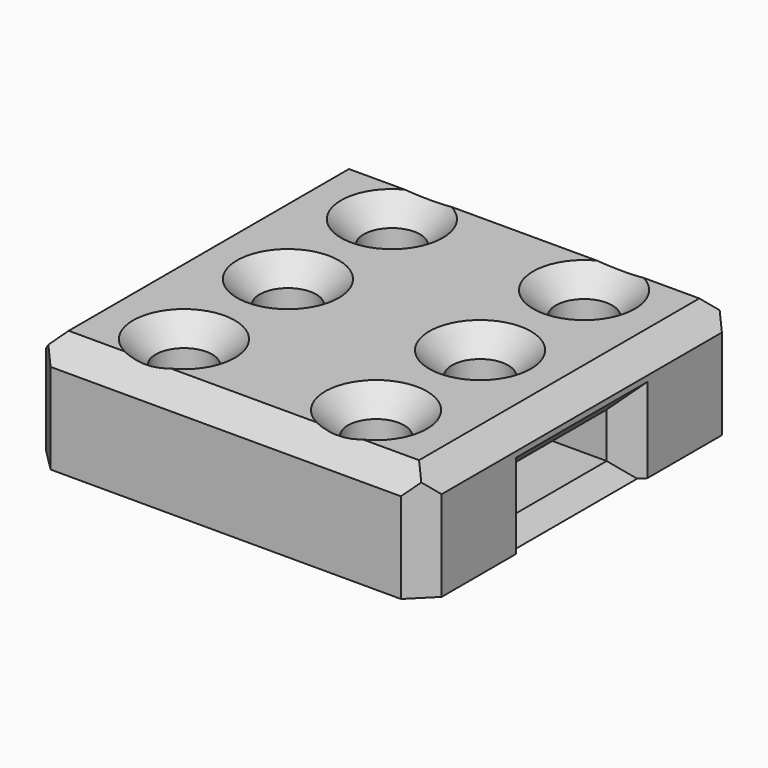
from build123d import *

# Parameters (mm, degrees)
F0_W          = 44.45
F0_H          = 44.45
F1_DEPTH      = 12.7
F2_W          = 13.335
F2_H          = 5.08
F3_DEPTH      = 76.2
F4_R          = 3.175
F5_DEPTH      = 25.4
F6_T1_DEPTH   = 57.5141495789
F6_T3_DEPTH   = 57.5141495789
F7_T1_DEPTH   = 5.08
F7_T3_DEPTH   = 13.335
F7_T5_DEPTH   = 23.2241495789
F7_T11_DEPTH  = 19.8670747894
F7_T16_DEPTH  = 11.6120747894
F7_T24_DEPTH  = 19.8670747894
F7_T28_DEPTH  = 11.6120747894
F7_T36_DEPTH  = 11.6120747894
F7_T41_DEPTH  = 19.8670747894
F7_T49_DEPTH  = 11.6120747894
F7_T54_DEPTH  = 19.8670747894
F7_T61_DEPTH  = 19.8670747894
F7_T65_DEPTH  = 11.6120747894
F7_T73_DEPTH  = 11.6120747894
F7_T78_DEPTH  = 19.8670747894
F7_T85_DEPTH  = 19.8670747894
F7_T90_DEPTH  = 11.6120747894
F7_T98_DEPTH  = 11.6120747894
F7_T103_DEPTH = 19.8670747894
F8_R          = 3.175
F9_DEPTH      = 1.905


# Not quite as in the source:
# - a fillet or chamfer that OpenCascade refuses, or shapes differently, is made with other operations: its cross-section is extruded or revolved along the edge and cut away or added


with BuildPart() as f1:
    # F0 (on Top) → F1 (new body)
    with BuildSketch(Plane.XY):
        Rectangle(F0_W, F0_H)
    extrude(amount=F1_DEPTH)

    # F2 (on face) → F3 (cut)
    with BuildSketch(Plane.YZ.offset(22.225)):
        with Locations((0, 4.445)):
            Rectangle(F2_W, F2_H)
    extrude(amount=-F3_DEPTH, mode=Mode.SUBTRACT)

    # F4 (on face) → F5 (cut)
    with BuildSketch(Plane.XY.offset(12.7)):
        with Locations((10.795, 14.605)):
            Circle(F4_R)
        with Locations((-10.795, 14.605)):
            Circle(F4_R)
        with Locations((-10.795, -14.605)):
            Circle(F4_R)
        with Locations((10.795, -14.605)):
            Circle(F4_R)
        with Locations((-10.795, 0)):
            Circle(F4_R)
        with Locations((10.795, 0)):
            Circle(F4_R)
    extrude(amount=-F5_DEPTH, mode=Mode.SUBTRACT)

    # F6: chamfer of 2.54 on 10 edges, made by hand

    # F6_s2 → F6_t1 (cut)
    with BuildSketch(Plane.XZ.offset(-28.7570747894)):
        Polygon((22.225, 10.16), (19.685, 12.7), (22.225, 12.7), align=None)
        Polygon((-19.685, 12.7), (-22.225, 10.16), (-22.225, 12.7), align=None)
    extrude(amount=F6_T1_DEPTH, mode=Mode.SUBTRACT)

    # F6_s4 → F6_t3 (cut)
    with BuildSketch(Plane.YZ.offset(-28.7570747894)):
        Polygon((-22.225, 10.16), (-19.685, 12.7), (-22.225, 12.7), align=None)
        Polygon((19.685, 12.7), (22.225, 10.16), (22.225, 12.7), align=None)
    extrude(amount=F6_T3_DEPTH, mode=Mode.SUBTRACT)

    # F6_s5 → F6_t6 (revolve, cut)
    with BuildSketch(Plane.XZ.offset(14.605)):
        Polygon((-5.08, 12.7), (-7.62, 10.16), (-7.62, 12.7), align=None)
    revolve(axis=Axis((-10.795, -14.605, 12.7), (0, 0, 1)), mode=Mode.SUBTRACT)

    # F6_s7 → F6_t8 (revolve, cut)
    with BuildSketch(Plane.XZ):
        Polygon((-5.08, 12.7), (-7.62, 10.16), (-7.62, 12.7), align=None)
    revolve(axis=Axis((-10.795, 0, 12.7), (0, 0, 1)), mode=Mode.SUBTRACT)

    # F6_s9 → F6_t10 (revolve, cut)
    with BuildSketch(Plane.XZ.offset(14.605)):
        Polygon((16.51, 12.7), (13.97, 10.16), (13.97, 12.7), align=None)
    revolve(axis=Axis((10.795, -14.605, 12.7), (0, 0, 1)), mode=Mode.SUBTRACT)

    # F6_s11 → F6_t12 (revolve, cut)
    with BuildSketch(Plane.XZ):
        Polygon((16.51, 12.7), (13.97, 10.16), (13.97, 12.7), align=None)
    revolve(axis=Axis((10.795, 0, 12.7), (0, 0, 1)), mode=Mode.SUBTRACT)

    # F6_s13 → F6_t14 (revolve, cut)
    with BuildSketch(Plane.XZ.offset(-14.605)):
        Polygon((-5.08, 12.7), (-7.62, 10.16), (-7.62, 12.7), align=None)
    revolve(axis=Axis((-10.795, 14.605, 12.7), (0, 0, 1)), mode=Mode.SUBTRACT)

    # F6_s15 → F6_t16 (revolve, cut)
    with BuildSketch(Plane.XZ.offset(-14.605)):
        Polygon((16.51, 12.7), (13.97, 10.16), (13.97, 12.7), align=None)
    revolve(axis=Axis((10.795, 14.605, 12.7), (0, 0, 1)), mode=Mode.SUBTRACT)

    # F7: chamfer of 2.54 on 12 edges, made by hand

    # F7_s2 → F7_t1 (cut)
    with BuildSketch(Plane.XY.offset(1.905)):
        Polygon((22.225, 9.2075), (19.685, 6.6675), (22.225, 6.6675), align=None)
        Polygon((22.225, -9.2075), (19.685, -6.6675), (22.225, -6.6675), align=None)
        Polygon((-19.685, 6.6675), (-22.225, 9.2075), (-22.225, 6.6675), align=None)
        Polygon((-19.685, -6.6675), (-22.225, -9.2075), (-22.225, -6.6675), align=None)
    extrude(amount=F7_T1_DEPTH, mode=Mode.SUBTRACT)

    # F7_s4 → F7_t3 (cut)
    with BuildSketch(Plane.XZ.offset(-6.6675)):
        Polygon((22.225, -0.635), (19.685, 1.905), (22.225, 1.905), align=None)
        Polygon((22.225, 9.525), (19.685, 6.985), (22.225, 6.985), align=None)
        Polygon((-19.685, 6.985), (-22.225, 9.525), (-22.225, 6.985), align=None)
        Polygon((-19.685, 1.905), (-22.225, -0.635), (-22.225, 1.905), align=None)
    extrude(amount=F7_T3_DEPTH, mode=Mode.SUBTRACT)

    # F7_s6 → F7_t5 (cut)
    with BuildSketch(Plane.XY.offset(-6.5320747894)):
        Polygon((-19.685, -22.225), (-22.225, -19.685), (-22.225, -22.225), align=None)
        Polygon((22.225, -19.685), (19.685, -22.225), (22.225, -22.225), align=None)
        Polygon((22.225, 19.685), (19.685, 22.225), (22.225, 22.225), align=None)
        Polygon((-19.685, 22.225), (-22.225, 19.685), (-22.225, 22.225), align=None)
    extrude(amount=F7_T5_DEPTH, mode=Mode.SUBTRACT)


with BuildPart() as f7_tool9:
    # F7_s10 → F7_t11 (new body)
    with BuildSketch(Plane.XZ.offset(6.6675)):
        Polygon((22.225, -0.635), (19.685, 1.905), (22.225, 1.905), align=None)
    extrude(amount=-F7_T11_DEPTH)

    split(bisect_by=Plane.XY, keep=Keep.TOP)

    split(bisect_by=Plane.XZ.offset(-6.6675), keep=Keep.BOTTOM)


with BuildPart() as f7_tool14:
    # F7_s15 → F7_t16 (new body)
    with BuildSketch(Plane.XY.offset(-4.6270747894)):
        Polygon((22.225, 9.2075), (19.685, 6.6675), (22.225, 6.6675), align=None)
    extrude(amount=F7_T16_DEPTH)

    split(bisect_by=Plane.XY, keep=Keep.TOP)

    split(bisect_by=Plane.XY.offset(1.905), keep=Keep.BOTTOM)


with BuildPart() as f7_tool9_1:
    add(f7_tool9.part)

    # F7_t19: intersect F7_tool14
    add(f7_tool14.part, mode=Mode.INTERSECT)


with BuildPart() as f1_1:
    add(f1.part)

    # F7_t7: cut F7_tool9
    add(f7_tool9_1.part, mode=Mode.SUBTRACT)


with BuildPart() as f7_tool22:
    # F7_s23 → F7_t24 (new body)
    with BuildSketch(Plane.XZ.offset(-13.1995747894)):
        Polygon((22.225, 9.525), (19.685, 6.985), (22.225, 6.985), align=None)
    extrude(amount=F7_T24_DEPTH)

    split(bisect_by=Plane.XZ.offset(-6.6675), keep=Keep.BOTTOM)


with BuildPart() as f7_tool26:
    # F7_s27 → F7_t28 (new body)
    with BuildSketch(Plane.XY.offset(1.905)):
        Polygon((22.225, 9.2075), (19.685, 6.6675), (22.225, 6.6675), align=None)
    extrude(amount=F7_T28_DEPTH)

    split(bisect_by=Plane(origin=(16.1925, 0, 16.1925), x_dir=(0, 1, 0), z_dir=(-0.7071067812, 0, -0.7071067812)), keep=Keep.TOP)

    split(bisect_by=Plane.XY.offset(6.985), keep=Keep.TOP)


with BuildPart() as f7_tool22_1:
    add(f7_tool22.part)

    # F7_t31: intersect F7_tool26
    add(f7_tool26.part, mode=Mode.INTERSECT)


with BuildPart() as f1_2:
    add(f1_1.part)

    # F7_t20: cut F7_tool22
    add(f7_tool22_1.part, mode=Mode.SUBTRACT)


with BuildPart() as f7_tool34:
    # F7_s35 → F7_t36 (new body)
    with BuildSketch(Plane.XY.offset(6.985)):
        Polygon((22.225, -9.2075), (19.685, -6.6675), (22.225, -6.6675), align=None)
    extrude(amount=-F7_T36_DEPTH)

    split(bisect_by=Plane.XY, keep=Keep.TOP)

    split(bisect_by=Plane.XY.offset(1.905), keep=Keep.BOTTOM)


with BuildPart() as f7_tool39:
    # F7_s40 → F7_t41 (new body)
    with BuildSketch(Plane.XZ.offset(13.1995747894)):
        Polygon((22.225, -0.635), (19.685, 1.905), (22.225, 1.905), align=None)
    extrude(amount=-F7_T41_DEPTH)

    split(bisect_by=Plane.XY, keep=Keep.TOP)

    split(bisect_by=Plane.XZ.offset(6.6675), keep=Keep.TOP)


with BuildPart() as f7_tool34_1:
    add(f7_tool34.part)

    # F7_t44: intersect F7_tool39
    add(f7_tool39.part, mode=Mode.INTERSECT)


with BuildPart() as f1_3:
    add(f1_2.part)

    # F7_t32: cut F7_tool34
    add(f7_tool34_1.part, mode=Mode.SUBTRACT)


with BuildPart() as f7_tool47:
    # F7_s48 → F7_t49 (new body)
    with BuildSketch(Plane.XY.offset(13.5170747894)):
        Polygon((22.225, -9.2075), (19.685, -6.6675), (22.225, -6.6675), align=None)
    extrude(amount=-F7_T49_DEPTH)

    split(bisect_by=Plane(origin=(16.1925, 0, 16.1925), x_dir=(0, 1, 0), z_dir=(-0.7071067812, 0, -0.7071067812)), keep=Keep.TOP)

    split(bisect_by=Plane.XY.offset(6.985), keep=Keep.TOP)


with BuildPart() as f7_tool52:
    # F7_s53 → F7_t54 (new body)
    with BuildSketch(Plane.XZ.offset(-6.6675)):
        Polygon((22.225, 9.525), (19.685, 6.985), (22.225, 6.985), align=None)
    extrude(amount=F7_T54_DEPTH)

    split(bisect_by=Plane.XZ.offset(6.6675), keep=Keep.TOP)


with BuildPart() as f7_tool47_1:
    add(f7_tool47.part)

    # F7_t56: intersect F7_tool52
    add(f7_tool52.part, mode=Mode.INTERSECT)


with BuildPart() as f1_4:
    add(f1_3.part)

    # F7_t45: cut F7_tool47
    add(f7_tool47_1.part, mode=Mode.SUBTRACT)


with BuildPart() as f7_tool59:
    # F7_s60 → F7_t61 (new body)
    with BuildSketch(Plane.XZ.offset(-13.1995747894)):
        Polygon((-19.685, 6.985), (-22.225, 9.525), (-22.225, 6.985), align=None)
    extrude(amount=F7_T61_DEPTH)

    split(bisect_by=Plane.XZ.offset(-6.6675), keep=Keep.BOTTOM)


with BuildPart() as f7_tool63:
    # F7_s64 → F7_t65 (new body)
    with BuildSketch(Plane.XY.offset(1.905)):
        Polygon((-19.685, 6.6675), (-22.225, 9.2075), (-22.225, 6.6675), align=None)
    extrude(amount=F7_T65_DEPTH)

    split(bisect_by=Plane.XY.offset(6.985), keep=Keep.TOP)

    split(bisect_by=Plane(origin=(-16.1925, 0, 16.1925), x_dir=(0, 1, 0), z_dir=(0.7071067812, 0, -0.7071067812)), keep=Keep.TOP)


with BuildPart() as f7_tool59_1:
    add(f7_tool59.part)

    # F7_t68: intersect F7_tool63
    add(f7_tool63.part, mode=Mode.INTERSECT)


with BuildPart() as f1_5:
    add(f1_4.part)

    # F7_t57: cut F7_tool59
    add(f7_tool59_1.part, mode=Mode.SUBTRACT)


with BuildPart() as f7_tool71:
    # F7_s72 → F7_t73 (new body)
    with BuildSketch(Plane.XY.offset(13.5170747894)):
        Polygon((-19.685, -6.6675), (-22.225, -9.2075), (-22.225, -6.6675), align=None)
    extrude(amount=-F7_T73_DEPTH)

    split(bisect_by=Plane.XY.offset(6.985), keep=Keep.TOP)

    split(bisect_by=Plane(origin=(-16.1925, 0, 16.1925), x_dir=(0, 1, 0), z_dir=(0.7071067812, 0, -0.7071067812)), keep=Keep.TOP)


with BuildPart() as f7_tool76:
    # F7_s77 → F7_t78 (new body)
    with BuildSketch(Plane.XZ.offset(-6.6675)):
        Polygon((-19.685, 6.985), (-22.225, 9.525), (-22.225, 6.985), align=None)
    extrude(amount=F7_T78_DEPTH)

    split(bisect_by=Plane.XZ.offset(6.6675), keep=Keep.TOP)


with BuildPart() as f7_tool71_1:
    add(f7_tool71.part)

    # F7_t80: intersect F7_tool76
    add(f7_tool76.part, mode=Mode.INTERSECT)


with BuildPart() as f1_6:
    add(f1_5.part)

    # F7_t69: cut F7_tool71
    add(f7_tool71_1.part, mode=Mode.SUBTRACT)


with BuildPart() as f7_tool83:
    # F7_s84 → F7_t85 (new body)
    with BuildSketch(Plane.XZ.offset(6.6675)):
        Polygon((-19.685, 1.905), (-22.225, -0.635), (-22.225, 1.905), align=None)
    extrude(amount=-F7_T85_DEPTH)

    split(bisect_by=Plane.XY, keep=Keep.TOP)

    split(bisect_by=Plane.XZ.offset(-6.6675), keep=Keep.BOTTOM)


with BuildPart() as f7_tool88:
    # F7_s89 → F7_t90 (new body)
    with BuildSketch(Plane.XY.offset(-4.6270747894)):
        Polygon((-19.685, 6.6675), (-22.225, 9.2075), (-22.225, 6.6675), align=None)
    extrude(amount=F7_T90_DEPTH)

    split(bisect_by=Plane.XY, keep=Keep.TOP)

    split(bisect_by=Plane.XY.offset(1.905), keep=Keep.BOTTOM)


with BuildPart() as f7_tool83_1:
    add(f7_tool83.part)

    # F7_t93: intersect F7_tool88
    add(f7_tool88.part, mode=Mode.INTERSECT)


with BuildPart() as f1_7:
    add(f1_6.part)

    # F7_t81: cut F7_tool83
    add(f7_tool83_1.part, mode=Mode.SUBTRACT)


with BuildPart() as f7_tool96:
    # F7_s97 → F7_t98 (new body)
    with BuildSketch(Plane.XY.offset(6.985)):
        Polygon((-19.685, -6.6675), (-22.225, -9.2075), (-22.225, -6.6675), align=None)
    extrude(amount=-F7_T98_DEPTH)

    split(bisect_by=Plane.XY, keep=Keep.TOP)

    split(bisect_by=Plane.XY.offset(1.905), keep=Keep.BOTTOM)


with BuildPart() as f7_tool101:
    # F7_s102 → F7_t103 (new body)
    with BuildSketch(Plane.XZ.offset(13.1995747894)):
        Polygon((-19.685, 1.905), (-22.225, -0.635), (-22.225, 1.905), align=None)
    extrude(amount=-F7_T103_DEPTH)

    split(bisect_by=Plane.XY, keep=Keep.TOP)

    split(bisect_by=Plane.XZ.offset(6.6675), keep=Keep.TOP)


with BuildPart() as f7_tool96_1:
    add(f7_tool96.part)

    # F7_t106: intersect F7_tool101
    add(f7_tool101.part, mode=Mode.INTERSECT)


with BuildPart() as f1_8:
    add(f1_7.part)

    # F7_t94: cut F7_tool96
    add(f7_tool96_1.part, mode=Mode.SUBTRACT)

    # F8 (on face) → F9 (join, through all)
    with BuildSketch(Plane(origin=(0, 0, 0), x_dir=(1, 0, 0), z_dir=(0, 0, -1))):
        with Locations((10.795, 0)):
            Circle(F8_R)
        with Locations((-10.795, 0)):
            Circle(F8_R)
    extrude(amount=-F9_DEPTH)


solid = f1_8.part
